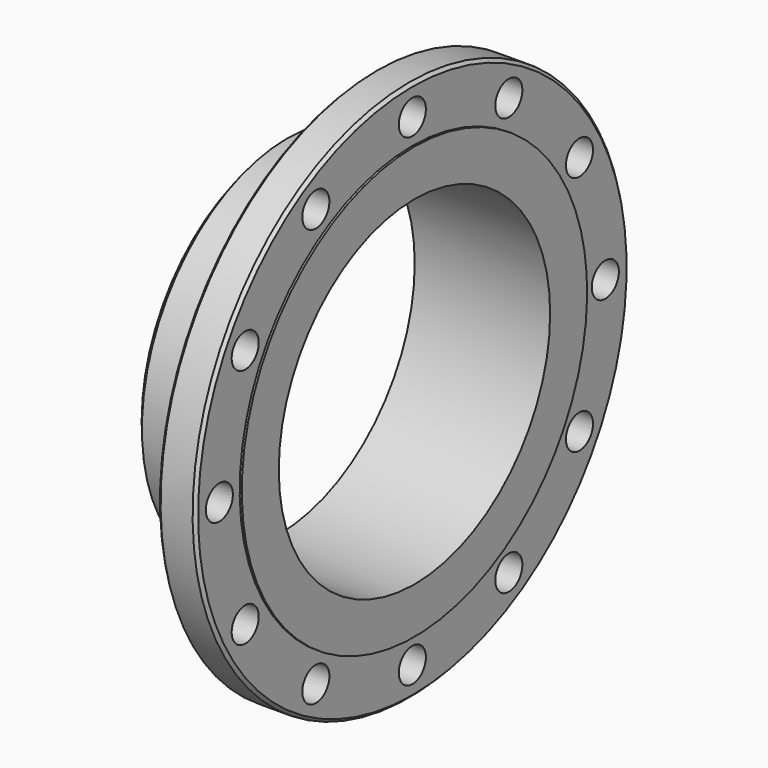
from build123d import *

# Parameters (mm, degrees)
F2_R            = 12.7
F3_DEPTH        = 30.1635
F3_COPIES_COUNT = 12
F4_R            = 3.175
F5_SIZE2        = 2.286
F5_SIZE         = 2.286


# Not quite as in the source:
# - a pattern or mirror of a feature is missing from the dataset's text; its kind, count and spacing are read off the source's solid


with BuildPart() as f1:
    # F0 (on Front) → F1 (revolve)
    with BuildSketch(Plane.XZ):
        Polygon((-101.6, 127.254), (0, 127.254), (0, 161.925), (-1.5875, 161.925), (-1.5875, 203.2), (-30.1625, 203.2), (-30.1625, 152.4), (-54.61, 138.1125), (-95.25, 136.525), (-101.6, 128.8415), align=None)
    revolve(axis=Axis((-71.3775697505, 0, 0), (-1, 0, 0)))

    # F2 (on face) → F3 (cut, through all)
    with BuildSketch(Plane(origin=(-30.1625, 0, 0), x_dir=(0, -1, 0), z_dir=(-1, 0, 0))):
        with Locations((0, 180.975)):
            Circle(F2_R)
    f3 = extrude(amount=-F3_DEPTH, mode=Mode.SUBTRACT)

    # F3_copies: F3 ×12 about axis
    f3_copies_axis = Axis((0, 0, 0), (1, 0, 0))
    for i in range(1, F3_COPIES_COUNT):
        add(f3.rotate(f3_copies_axis, i * 360 / F3_COPIES_COUNT), mode=Mode.SUBTRACT)

    # F4
    f4_edges = [f1.edges().sort_by_distance(p)[0] for p in [
        (-30.1625, 0, -152.4),
        (-54.61, 0, -138.1125),
    ]]
    fillet(f4_edges, radius=F4_R)

    # F5
    f5_edges = [f1.edges().sort_by_distance(p)[0] for p in [
        (-1.5875, 0, -203.2),
        (-30.1625, 0, -203.2),
        (-15.875, 0, 203.2),
    ]]
    chamfer(f5_edges, length=F5_SIZE, length2=F5_SIZE2)


solid = f1.part
